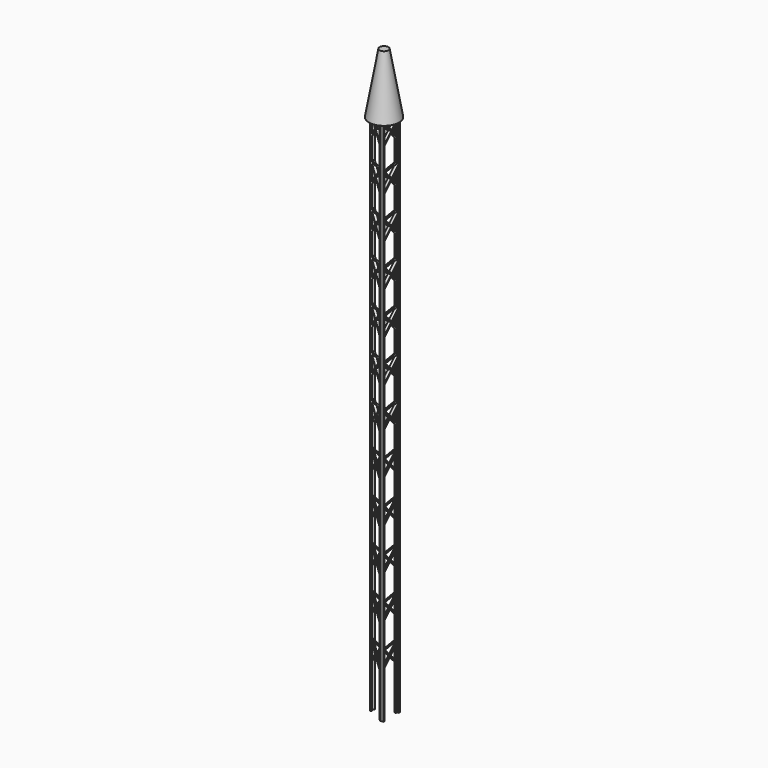
from build123d import *

# Parameters (mm, degrees)
F1_DEPTH = 25.4
F2_DEPTH = 25.4
F3_DEPTH = 25.4
F5_COUNT = 2
F5_ANGLE = 60
F6_COUNT = 2
F6_ANGLE = 60
F7_R     = 254
F8_DEPTH = 1016
F8_TAPER = 10


# Not quite as in the source:
# - a feature names something its author has since deleted; it is built from what else it names


with BuildPart() as f1:
    # F0 (on Right) → F1 (new body)
    with BuildSketch(Plane.YZ):
        Polygon((177.8, 1676.4), (25.4, 1828.8), (25.4, 1803.4), (165.1, 1663.7), align=None)
        Polygon((25.4, 1828.8), (0, 1828.8), (0, -7061.2), (25.4, -7061.2), (25.4, -6324.6), (25.4, -6299.2), (25.4, -6019.8), (25.4, -5994.4), (25.4, -5613.4), (25.4, -5588), (25.4, -5308.6), (25.4, -5283.2), (25.4, -4902.2), (25.4, -4876.8), (25.4, -4597.4), (25.4, -4572), (25.4, -4191), (25.4, -4165.6), (25.4, -3886.2), (25.4, -3860.8), (25.4, -3479.8), (25.4, -3454.4), (25.4, -3175), (25.4, -3149.6), (25.4, -2768.6), (25.4, -2743.2), (25.4, -2463.8), (25.4, -2438.4), (25.4, -2057.4), (25.4, -2032), (25.4, -1752.6), (25.4, -1727.2), (25.4, -1346.2), (25.4, -1320.8), (25.4, -1041.4), (25.4, -1016), (25.4, -635), (25.4, -609.6), (25.4, -330.2), (25.4, -304.8), (25.4, 76.2), (25.4, 101.6), (25.4, 381), (25.4, 406.4), (25.4, 787.4), (25.4, 812.8), (25.4, 1092.2), (25.4, 1117.6), (25.4, 1498.6), (25.4, 1524), (25.4, 1803.4), align=None)
        Polygon((165.1, 952.5), (177.8, 965.2), (25.4, 1117.6), (25.4, 1092.2), align=None)
        Polygon((177.8, 939.8), (177.8, 965.2), (165.1, 952.5), align=None)
        Polygon((190.5, 952.5), (177.8, 965.2), (177.8, 939.8), align=None)
        Polygon((330.2, 812.8), (190.5, 952.5), (177.8, 939.8), (330.2, 787.4), align=None)
        Polygon((177.8, 1651), (177.8, 1676.4), (165.1, 1663.7), align=None)
        Polygon((190.5, 1663.7), (177.8, 1676.4), (177.8, 1651), align=None)
        Polygon((330.2, 1524), (190.5, 1663.7), (177.8, 1651), (330.2, 1498.6), align=None)
        Polygon((355.6, 1828.8), (330.2, 1828.8), (330.2, 1803.4), (330.2, 1524), (330.2, 1498.6), (330.2, 1117.6), (330.2, 1092.2), (330.2, 812.8), (330.2, 787.4), (330.2, 406.4), (330.2, 381), (330.2, 101.6), (330.2, 76.2), (330.2, -304.8), (330.2, -330.2), (330.2, -609.6), (330.2, -635), (330.2, -1016), (330.2, -1041.4), (330.2, -1320.8), (330.2, -1346.2), (330.2, -1727.2), (330.2, -1752.6), (330.2, -2032), (330.2, -2057.4), (330.2, -2438.4), (330.2, -2463.8), (330.2, -2743.2), (330.2, -2768.6), (330.2, -3149.6), (330.2, -3175), (330.2, -3454.4), (330.2, -3479.8), (330.2, -3860.8), (330.2, -3886.2), (330.2, -4165.6), (330.2, -4191), (330.2, -4572), (330.2, -4597.4), (330.2, -4876.8), (330.2, -4902.2), (330.2, -5283.2), (330.2, -5308.6), (330.2, -5588), (330.2, -5613.4), (330.2, -5994.4), (330.2, -6019.8), (330.2, -6299.2), (330.2, -6324.6), (330.2, -7061.2), (355.6, -7061.2), align=None)
        Polygon((165.1, 241.3), (177.8, 254), (25.4, 406.4), (25.4, 381), align=None)
        Polygon((330.2, 101.6), (190.5, 241.3), (177.8, 228.6), (330.2, 76.2), align=None)
        Polygon((165.1, 1663.7), (25.4, 1524), (25.4, 1498.6), (177.8, 1651), align=None)
        Polygon((177.8, -457.2), (25.4, -304.8), (25.4, -330.2), (165.1, -469.9), align=None)
        Polygon((330.2, -635), (330.2, -609.6), (190.5, -469.9), (177.8, -482.6), align=None)
        Polygon((190.5, -469.9), (177.8, -457.2), (165.1, -469.9), (177.8, -482.6), align=None)
        Polygon((25.4, 787.4), (177.8, 939.8), (165.1, 952.5), (25.4, 812.8), align=None)
        Polygon((177.8, 228.6), (177.8, 254), (165.1, 241.3), align=None)
        Polygon((190.5, 241.3), (177.8, 254), (177.8, 228.6), align=None)
        Polygon((330.2, 1828.8), (177.8, 1676.4), (190.5, 1663.7), (330.2, 1803.4), align=None)
        Polygon((330.2, 1117.6), (177.8, 965.2), (190.5, 952.5), (330.2, 1092.2), align=None)
        Polygon((330.2, 406.4), (177.8, 254), (190.5, 241.3), (330.2, 381), align=None)
        Polygon((330.2, -330.2), (330.2, -304.8), (177.8, -457.2), (190.5, -469.9), align=None)
        Polygon((177.8, -1168.4), (25.4, -1016), (25.4, -1041.4), (165.1, -1181.1), align=None)
        Polygon((330.2, -1346.2), (330.2, -1320.8), (190.5, -1181.1), (177.8, -1193.8), align=None)
        Polygon((190.5, -1181.1), (177.8, -1168.4), (165.1, -1181.1), (177.8, -1193.8), align=None)
        Polygon((25.4, 76.2), (177.8, 228.6), (165.1, 241.3), (25.4, 101.6), align=None)
        Polygon((330.2, -1041.4), (330.2, -1016), (177.8, -1168.4), (190.5, -1181.1), align=None)
        Polygon((330.2, -1752.6), (330.2, -1727.2), (177.8, -1879.6), (190.5, -1892.3), align=None)
        Polygon((330.2, -2463.8), (330.2, -2438.4), (177.8, -2590.8), (190.5, -2603.5), align=None)
        Polygon((177.8, -1879.6), (25.4, -1727.2), (25.4, -1752.6), (165.1, -1892.3), align=None)
        Polygon((330.2, -2057.4), (330.2, -2032), (190.5, -1892.3), (177.8, -1905), align=None)
        Polygon((190.5, -1892.3), (177.8, -1879.6), (165.1, -1892.3), (177.8, -1905), align=None)
        Polygon((177.8, -482.6), (165.1, -469.9), (25.4, -609.6), (25.4, -635), align=None)
        Polygon((177.8, -2590.8), (25.4, -2438.4), (25.4, -2463.8), (165.1, -2603.5), align=None)
        Polygon((330.2, -2768.6), (330.2, -2743.2), (190.5, -2603.5), (177.8, -2616.2), align=None)
        Polygon((190.5, -2603.5), (177.8, -2590.8), (165.1, -2603.5), (177.8, -2616.2), align=None)
        Polygon((177.8, -1193.8), (165.1, -1181.1), (25.4, -1320.8), (25.4, -1346.2), align=None)
        Polygon((177.8, -1905), (165.1, -1892.3), (25.4, -2032), (25.4, -2057.4), align=None)
    extrude(amount=F1_DEPTH)

    # F0 (on Right) + F1_face (on face) → F2 (join)
    with BuildSketch(Plane.YZ):
        Polygon((190.5, -1892.3), (177.8, -1879.6), (165.1, -1892.3), (177.8, -1905), align=None)
        Polygon((177.8, -1905), (165.1, -1892.3), (25.4, -2032), (25.4, -2057.4), align=None)
        Polygon((25.4, -3149.6), (25.4, -3175), (165.1, -3314.7), (177.8, -3302), align=None)
        Polygon((190.5, -2603.5), (177.8, -2590.8), (165.1, -2603.5), (177.8, -2616.2), align=None)
        Polygon((330.2, -2057.4), (330.2, -2032), (190.5, -1892.3), (177.8, -1905), align=None)
        Polygon((177.8, -3302), (190.5, -3314.7), (330.2, -3175), (330.2, -3149.6), align=None)
        Polygon((165.1, -3314.7), (177.8, -3327.4), (190.5, -3314.7), (177.8, -3302), align=None)
        Polygon((190.5, -3314.7), (177.8, -3327.4), (330.2, -3479.8), (330.2, -3454.4), align=None)
        Polygon((177.8, -4724.4), (190.5, -4737.1), (330.2, -4597.4), (330.2, -4572), align=None)
        Polygon((330.2, -2768.6), (330.2, -2743.2), (190.5, -2603.5), (177.8, -2616.2), align=None)
        Polygon((177.8, -4013.2), (190.5, -4025.9), (330.2, -3886.2), (330.2, -3860.8), align=None)
        Polygon((177.8, -2616.2), (165.1, -2603.5), (25.4, -2743.2), (25.4, -2768.6), align=None)
        Polygon((25.4, -3860.8), (25.4, -3886.2), (165.1, -4025.9), (177.8, -4013.2), align=None)
        Polygon((25.4, -3454.4), (25.4, -3479.8), (177.8, -3327.4), (165.1, -3314.7), align=None)
        Polygon((25.4, -4572), (25.4, -4597.4), (165.1, -4737.1), (177.8, -4724.4), align=None)
        Polygon((165.1, -4025.9), (177.8, -4038.6), (190.5, -4025.9), (177.8, -4013.2), align=None)
        Polygon((190.5, -4025.9), (177.8, -4038.6), (330.2, -4191), (330.2, -4165.6), align=None)
        Polygon((177.8, -5435.6), (190.5, -5448.3), (330.2, -5308.6), (330.2, -5283.2), align=None)
        Polygon((25.4, -4165.6), (25.4, -4191), (177.8, -4038.6), (165.1, -4025.9), align=None)
        Polygon((25.4, -5283.2), (25.4, -5308.6), (165.1, -5448.3), (177.8, -5435.6), align=None)
        Polygon((25.4, -4876.8), (25.4, -4902.2), (177.8, -4749.8), (165.1, -4737.1), align=None)
    with BuildSketch(Plane(origin=(25.4, 178.3311693353, -2204.6127802038), x_dir=(0, 1, 0), z_dir=(1, 0, 0))):
        Polygon((-152.9311693353, -259.1872197962), (151.8688306647, -563.9872197962), (151.8688306647, -4856.5872197962), (177.2688306647, -4856.5872197962), (177.2688306647, 4033.4127802038), (151.8688306647, 4033.4127802038), (-0.5311693353, 3881.0127802038), (-152.9311693353, 4033.4127802038), (-178.3311693353, 4033.4127802038), (-178.3311693353, -4856.5872197962), (-152.9311693353, -4856.5872197962), align=None)
        Polygon((-152.9311693353, 172.6127802038), (-152.9311693353, 452.0127802038), (-13.2311693353, 312.3127802038), align=None, mode=Mode.SUBTRACT)
        Polygon((-152.9311693353, 883.8127802038), (-152.9311693353, 1163.2127802038), (-13.2311693353, 1023.5127802038), align=None, mode=Mode.SUBTRACT)
        Polygon((-13.2311693353, 1734.7127802038), (-152.9311693353, 1595.0127802038), (-152.9311693353, 1874.4127802038), align=None, mode=Mode.SUBTRACT)
        Polygon((151.8688306647, -233.7872197962), (-0.5311693353, -386.1872197962), (-152.9311693353, -233.7872197962), (-152.9311693353, 147.2127802038), (-0.5311693353, 299.6127802038), (151.8688306647, 147.2127802038), align=None, mode=Mode.SUBTRACT)
        Polygon((151.8688306647, -538.5872197962), (12.1688306647, -398.8872197962), (151.8688306647, -259.1872197962), align=None, mode=Mode.SUBTRACT)
        Polygon((151.8688306647, 172.6127802038), (12.1688306647, 312.3127802038), (151.8688306647, 452.0127802038), align=None, mode=Mode.SUBTRACT)
        Polygon((151.8688306647, 477.4127802038), (-0.5311693353, 325.0127802038), (-152.9311693353, 477.4127802038), (-152.9311693353, 858.4127802038), (-0.5311693353, 1010.8127802038), (151.8688306647, 858.4127802038), align=None, mode=Mode.SUBTRACT)
        Polygon((-152.9311693353, 1569.6127802038), (-0.5311693353, 1722.0127802038), (151.8688306647, 1569.6127802038), (151.8688306647, 1188.6127802038), (-0.5311693353, 1036.2127802038), (-152.9311693353, 1188.6127802038), align=None, mode=Mode.SUBTRACT)
        Polygon((151.8688306647, 1163.2127802038), (151.8688306647, 883.8127802038), (12.1688306647, 1023.5127802038), align=None, mode=Mode.SUBTRACT)
        Polygon((-152.9311693353, 2585.6127802038), (-13.2311693353, 2445.9127802038), (-152.9311693353, 2306.2127802038), align=None, mode=Mode.SUBTRACT)
        Polygon((151.8688306647, 1899.8127802038), (-0.5311693353, 1747.4127802038), (-152.9311693353, 1899.8127802038), (-152.9311693353, 2280.8127802038), (-0.5311693353, 2433.2127802038), (151.8688306647, 2280.8127802038), align=None, mode=Mode.SUBTRACT)
        Polygon((-152.9311693353, 3017.4127802038), (-152.9311693353, 3296.8127802038), (-13.2311693353, 3157.1127802038), align=None, mode=Mode.SUBTRACT)
        Polygon((-152.9311693353, 3728.6127802038), (-152.9311693353, 4008.0127802038), (-13.2311693353, 3868.3127802038), align=None, mode=Mode.SUBTRACT)
        Polygon((-0.5311693353, 2458.6127802038), (-152.9311693353, 2611.0127802038), (-152.9311693353, 2992.0127802038), (-0.5311693353, 3144.4127802038), (151.8688306647, 2992.0127802038), (151.8688306647, 2611.0127802038), align=None, mode=Mode.SUBTRACT)
        Polygon((151.8688306647, 1595.0127802038), (12.1688306647, 1734.7127802038), (151.8688306647, 1874.4127802038), align=None, mode=Mode.SUBTRACT)
        Polygon((151.8688306647, 2306.2127802038), (12.1688306647, 2445.9127802038), (151.8688306647, 2585.6127802038), align=None, mode=Mode.SUBTRACT)
        Polygon((-0.5311693353, 3169.8127802038), (-152.9311693353, 3322.2127802038), (-152.9311693353, 3703.2127802038), (-0.5311693353, 3855.6127802038), (151.8688306647, 3703.2127802038), (151.8688306647, 3322.2127802038), align=None, mode=Mode.SUBTRACT)
        Polygon((151.8688306647, 3017.4127802038), (12.1688306647, 3157.1127802038), (151.8688306647, 3296.8127802038), align=None, mode=Mode.SUBTRACT)
        Polygon((151.8688306647, 4008.0127802038), (151.8688306647, 3728.6127802038), (12.1688306647, 3868.3127802038), align=None, mode=Mode.SUBTRACT)
    extrude(amount=F2_DEPTH)

    # F0 (on Right) → F3 (join)
    with BuildSketch(Plane.YZ):
        Polygon((25.4, -5994.4), (25.4, -6019.8), (165.1, -6159.5), (177.8, -6146.8), align=None)
        Polygon((165.1, -6159.5), (177.8, -6172.2), (190.5, -6159.5), (177.8, -6146.8), align=None)
        Polygon((190.5, -6159.5), (177.8, -6172.2), (330.2, -6324.6), (330.2, -6299.2), align=None)
        Polygon((190.5, -5448.3), (177.8, -5461), (330.2, -5613.4), (330.2, -5588), align=None)
        Polygon((165.1, -5448.3), (177.8, -5461), (190.5, -5448.3), (177.8, -5435.6), align=None)
        Polygon((165.1, -4737.1), (177.8, -4749.8), (190.5, -4737.1), (177.8, -4724.4), align=None)
        Polygon((190.5, -4737.1), (177.8, -4749.8), (330.2, -4902.2), (330.2, -4876.8), align=None)
        Polygon((25.4, -4876.8), (25.4, -4902.2), (177.8, -4749.8), (165.1, -4737.1), align=None)
        Polygon((25.4, -5588), (25.4, -5613.4), (177.8, -5461), (165.1, -5448.3), align=None)
        Polygon((177.8, -6146.8), (190.5, -6159.5), (330.2, -6019.8), (330.2, -5994.4), align=None)
        Polygon((25.4, -6299.2), (25.4, -6324.6), (177.8, -6172.2), (165.1, -6159.5), align=None)
    extrude(amount=F3_DEPTH)


with BuildPart() as f5_1:
    # F5: instance of F1
    add(f1.part.rotate(Axis((0, 0, 0), (0, 0, 1)), 1 * F5_ANGLE / (F5_COUNT - 1)))


with BuildPart() as f6_1:
    # F6: instance of F1
    add(f1.part.rotate(Axis((0, 355.6, 0), (0, 0, -1)), 1 * F6_ANGLE / (F6_COUNT - 1)))


with BuildPart() as f1_1:
    add(f1.part)

    add(f5_1.part)  # F8 merges F5_1

    add(f6_1.part)  # F8 merges F6_1
    # F7 (on face) → F8 (join)
    with BuildSketch(Plane.XY.offset(1828.8)):
        with Locations((-79.3586335857, 177.8)):
            Circle(F7_R)
    extrude(amount=F8_DEPTH, taper=F8_TAPER)


solid = f1_1.part
